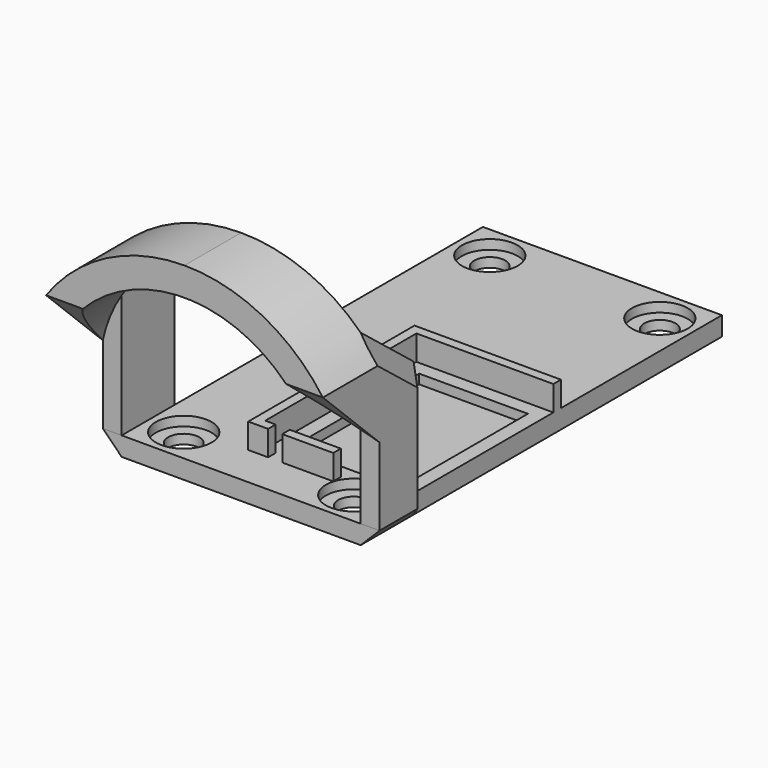
from build123d import *

# Parameters (mm, degrees)
F0_R      = 1.65
F1_DEPTH  = 2
F2_R      = 2.95
F2_R_2    = 1.65
F2_W      = 11.5
F2_H      = 17
F3_DEPTH  = 1
F4_W      = 5.4
F4_H      = 1
F5_DEPTH  = 2.65
F7_DEPTH  = 23
F9_DEPTH  = 7.5
F10_DEPTH = 55.301
F12_DEPTH = 29.301
F13_SIZE  = 1.99999
F15_DEPTH = 2.001
F17_DEPTH = 2.001
F18_SIZE  = 1.99999


# Not quite as in the source:
# - a fillet or chamfer is up to 0.001 mm smaller than in the source, because OpenCascade refuses the exact size


with BuildPart() as f1:
    # F0 (on Top) → F1 (new body)
    with BuildSketch(Plane.XY):
        Polygon((2.8630541071, 32.0832646102), (-22.4369458929, 32.0832646102), (-22.4369458929, -8.7167353898), (-24.4369458929, -10.7167353898), (-24.4369458929, -15.7167353898), (-21.1369458929, -15.7167353898), (2.8630541071, -15.7167353898), (4.8630541071, -15.7167353898), (4.8630541071, -10.7167353898), (2.8630541071, -8.7167353898), align=None)
        with Locations((-18.7869458929, -12.0667353898)):
            Circle(F0_R, mode=Mode.SUBTRACT)
        with Locations((-0.7869458929, -12.0667353898)):
            Circle(F0_R, mode=Mode.SUBTRACT)
        with Locations((-18.7869458929, 28.4332646102)):
            Circle(F0_R, mode=Mode.SUBTRACT)
        with Locations((-0.7869458929, 28.4332646102)):
            Circle(F0_R, mode=Mode.SUBTRACT)
    extrude(amount=F1_DEPTH)

    # F2 (on face) → F3 (cut)
    with BuildSketch(Plane.XY.offset(2)):
        with Locations((-18.7869458929, -12.0667353898)):
            Circle(F2_R)
        with Locations((-18.7869458929, -12.0667353898)):
            Circle(F2_R_2, mode=Mode.SUBTRACT)
        with Locations((-0.7869458929, -12.0667353898)):
            Circle(F2_R)
        with Locations((-0.7869458929, -12.0667353898)):
            Circle(F2_R_2, mode=Mode.SUBTRACT)
        with Locations((-18.7869458929, 28.4332646102)):
            Circle(F2_R)
        with Locations((-18.7869458929, 28.4332646102)):
            Circle(F2_R_2, mode=Mode.SUBTRACT)
        with Locations((-0.7869458929, 28.4332646102)):
            Circle(F2_R)
        with Locations((-0.7869458929, 28.4332646102)):
            Circle(F2_R_2, mode=Mode.SUBTRACT)
        with Locations((-4.3869458929, -0.2167353898)):
            Rectangle(F2_W, F2_H)
    extrude(amount=-F3_DEPTH, mode=Mode.SUBTRACT)

    # F4 (on face) → F5 (join)
    with BuildSketch(Plane.XY.offset(2)):
        Polygon((-10.5369458929, -11.2167353898), (-10.5369458929, -10.2167353898), (-11.6369458929, -10.2167353898), (-11.6369458929, 9.7832646102), (2.8630541071, 9.7832646102), (2.8630541071, 10.7832646102), (-12.6369458929, 10.7832646102), (-12.6369458929, -11.2167353898), align=None)
        with Locations((-6.3369458929, -10.7167353898)):
            Rectangle(F4_W, F4_H)
    extrude(amount=F5_DEPTH)

    # F13 (size 2 in the source; OpenCascade refuses exactly that, so slightly less here)
    f13_edges = [f1.edges().sort_by_distance(p)[0] for p in [
        (4.863054, -13.216735, 0),
        (-24.436946, -13.216735, 0),
    ]]
    chamfer(f13_edges, length=F13_SIZE)


with BuildPart() as f7:
    # F6 (on face) → F7 (new body)
    with BuildSketch(Plane.XY.offset(2)):
        Polygon((4.8630541071, -15.7167353898), (2.8630541071, -15.7167353898), (-22.4369458929, -15.7167353898), (-24.4369458929, -15.7167353898), (-24.4369458929, -23.2167353898), (4.8630541071, -23.2167353898), align=None)
        Polygon((4.8630541071, -10.7167353898), (2.8630541071, -8.7167353898), (2.8630541071, -15.7167353898), (4.8630541071, -15.7167353898), align=None)
        Polygon((-24.4369458929, -15.7167353898), (-22.4369458929, -15.7167353898), (-22.4369458929, -8.7167353898), (-24.4369458929, -10.7167353898), align=None)
    extrude(amount=F7_DEPTH)

    # F8 (on face) → F9 (cut)
    with BuildSketch(Plane.XZ.offset(23.2167353898)):
        with BuildLine():
            Line((4.8630541071, 2), (4.8630541071, 10.2214127336))
            ThreePointArc((4.8630541071, 10.2214127336), (-9.7869458929, 22), (-24.4369458929, 10.2214127336))
            Line((-24.4369458929, 10.2214127336), (-24.4369458929, 2))
            Line((-24.4369458929, 2), (4.8630541071, 2))
        make_face()
    extrude(amount=-F9_DEPTH, mode=Mode.SUBTRACT)

    # F8 (on face) → F10 (cut, through all)
    with BuildSketch(Plane.XZ.offset(23.2167353898)):
        with BuildLine():
            Line((-24.4369458929, 25), (-24.4369458929, 17.4583698539))
            ThreePointArc((-24.4369458929, 17.4583698539), (-18.0255544717, 23.0039160422), (-9.7869458929, 25))
            Line((-9.7869458929, 25), (-24.4369458929, 25))
        make_face()
        with BuildLine():
            ThreePointArc((-9.7869458929, 25), (-1.548337314, 23.0039160422), (4.8630541071, 17.4583698539))
            Line((4.8630541071, 17.4583698539), (4.8630541071, 25))
            Line((4.8630541071, 25), (-9.7869458929, 25))
        make_face()
    extrude(amount=-F10_DEPTH, mode=Mode.SUBTRACT)

    # F11 (on face) → F12 (cut, through all)
    with BuildSketch(Plane.YZ.offset(4.8630541071)):
        Polygon((-23.2167353898, 10.2214127336), (-15.7167353898, 10.2214127336), (-23.2167353898, 17.4583698539), align=None)
    extrude(amount=-F12_DEPTH, mode=Mode.SUBTRACT)

    # F14 (on face) → F15 (cut, through all)
    with BuildSketch(Plane.YZ.offset(-22.4369458929)):
        Polygon((-8.7167353898, 19.8053699673), (-15.7167353898, 19.8053699673), (-8.7167353898, 14.2720625306), align=None)
    extrude(amount=-F15_DEPTH, mode=Mode.SUBTRACT)

    # F16 (on face) → F17 (cut, through all)
    with BuildSketch(Plane(origin=(2.8630541071, 0, 0), x_dir=(0, -1, 0), z_dir=(-1, 0, 0))):
        Polygon((15.7167353898, 19.8053699673), (8.7167353898, 19.8053699673), (8.7167353898, 14.2720625306), align=None)
    extrude(amount=-F17_DEPTH, mode=Mode.SUBTRACT)

    # F18 (size 2 in the source; OpenCascade refuses exactly that, so slightly less here)
    f18_edges = [f7.edges().sort_by_distance(p)[0] for p in [
        (-24.436946, -11.73218, 16.655689),
        (4.863054, -11.73218, 16.655689),
    ]]
    chamfer(f18_edges, length=F18_SIZE)


solid = Compound([f1.part, f7.part])
